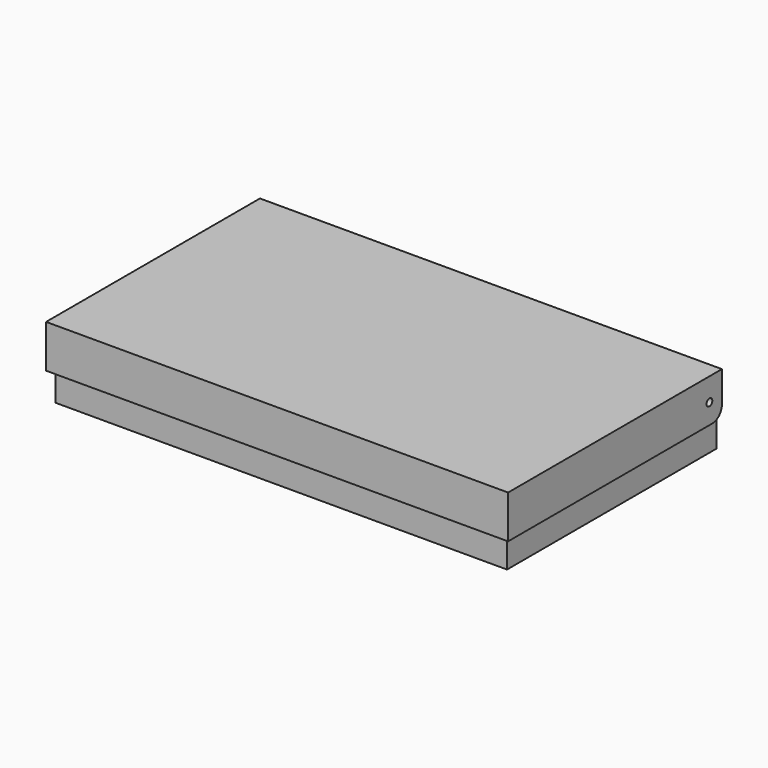
from build123d import *

# Parameters (mm, degrees)
F0_W          = 189.0018912738
F0_H          = 109.5
F0_W_2        = 25
F0_H_2        = 25
F1_DEPTH      = 25
F2_W          = 189.0018912738
F2_H          = 109.5
F3_DEPTH      = 2
F4_R          = 15
F6_DEPTH      = 3
F6_DEPTH_BACK = 15
F7_W          = 193.4018912738
F7_H          = 111.8995610192
F8_DEPTH      = 2
F9_T1_DEPTH   = 204.0018912738
F10_R         = 1.5
F11_DEPTH     = 200
F12_R         = 5


# Not quite as in the source:
# - a fillet or chamfer that OpenCascade refuses, or shapes differently, is made with other operations: its cross-section is extruded or revolved along the edge and cut away or added


with BuildPart() as f1:
    # F0 (on Top) → F1 (new body)
    with BuildSketch(Plane.XY):
        with Locations((79.4990543631, -39.75)):
            Rectangle(F0_W, F0_H)
        with Locations((0.0173321555, -79.5)):
            Rectangle(F0_W_2, F0_H_2, mode=Mode.SUBTRACT)
        with Locations((26.5173321555, -79.5)):
            Rectangle(F0_W_2, F0_H_2, mode=Mode.SUBTRACT)
        with Locations((53.0173321555, -79.5)):
            Rectangle(F0_W_2, F0_H_2, mode=Mode.SUBTRACT)
        with Locations((-0.0018912738, -53)):
            Rectangle(F0_W_2, F0_H_2, mode=Mode.SUBTRACT)
        with Locations((26.4981087262, -53)):
            Rectangle(F0_W_2, F0_H_2, mode=Mode.SUBTRACT)
        with Locations((52.9981087262, -53)):
            Rectangle(F0_W_2, F0_H_2, mode=Mode.SUBTRACT)
        with Locations((79.4981087262, -53)):
            Rectangle(F0_W_2, F0_H_2, mode=Mode.SUBTRACT)
        with Locations((79.5173321555, -79.5)):
            Rectangle(F0_W_2, F0_H_2, mode=Mode.SUBTRACT)
        with Locations((106.0173321555, -79.5)):
            Rectangle(F0_W_2, F0_H_2, mode=Mode.SUBTRACT)
        with Locations((132.5173321555, -79.5)):
            Rectangle(F0_W_2, F0_H_2, mode=Mode.SUBTRACT)
        with Locations((159.0173321555, -79.5)):
            Rectangle(F0_W_2, F0_H_2, mode=Mode.SUBTRACT)
        with Locations((105.9981087262, -53)):
            Rectangle(F0_W_2, F0_H_2, mode=Mode.SUBTRACT)
        with Locations((132.4981087262, -53)):
            Rectangle(F0_W_2, F0_H_2, mode=Mode.SUBTRACT)
        with Locations((158.9981087262, -53)):
            Rectangle(F0_W_2, F0_H_2, mode=Mode.SUBTRACT)
        with Locations((-0.0081907397, -26.5)):
            Rectangle(F0_W_2, F0_H_2, mode=Mode.SUBTRACT)
        with Locations((26.4918092603, -26.5)):
            Rectangle(F0_W_2, F0_H_2, mode=Mode.SUBTRACT)
        with Locations((52.9918092603, -26.5)):
            Rectangle(F0_W_2, F0_H_2, mode=Mode.SUBTRACT)
        with Locations((79.4918092603, -26.5)):
            Rectangle(F0_W_2, F0_H_2, mode=Mode.SUBTRACT)
        Rectangle(F0_W_2, F0_H_2, mode=Mode.SUBTRACT)
        with Locations((26.5, 0)):
            Rectangle(F0_W_2, F0_H_2, mode=Mode.SUBTRACT)
        with Locations((53, 0)):
            Rectangle(F0_W_2, F0_H_2, mode=Mode.SUBTRACT)
        with Locations((105.9918092603, -26.5)):
            Rectangle(F0_W_2, F0_H_2, mode=Mode.SUBTRACT)
        with Locations((132.4918092603, -26.5)):
            Rectangle(F0_W_2, F0_H_2, mode=Mode.SUBTRACT)
        with Locations((158.9918092603, -26.5)):
            Rectangle(F0_W_2, F0_H_2, mode=Mode.SUBTRACT)
        with Locations((79.5, 0)):
            Rectangle(F0_W_2, F0_H_2, mode=Mode.SUBTRACT)
        with Locations((106, 0)):
            Rectangle(F0_W_2, F0_H_2, mode=Mode.SUBTRACT)
        with Locations((132.5, 0)):
            Rectangle(F0_W_2, F0_H_2, mode=Mode.SUBTRACT)
        with Locations((159, 0)):
            Rectangle(F0_W_2, F0_H_2, mode=Mode.SUBTRACT)
    extrude(amount=F1_DEPTH)

    # F2 (on Top) → F3 (join)
    with BuildSketch(Plane.XY):
        with Locations((79.4990543631, -39.75)):
            Rectangle(F2_W, F2_H)
    extrude(amount=-F3_DEPTH)

    # F4
    f4_edges = [f1.edges().sort_by_distance(p)[0] for p in [
        (0, -12.5, 0),
        (26.5, -12.5, 0),
        (53, -12.5, 0),
        (79.5, -12.5, 0),
        (106, -12.5, 0),
        (132.5, -12.5, 0),
        (159, -12.5, 0),
        (-0.008191, -39, 0),
        (26.491809, -39, 0),
        (52.991809, -39, 0),
        (79.491809, -39, 0),
        (105.991809, -39, 0),
        (132.491809, -39, 0),
        (158.991809, -39, 0),
        (158.998109, -65.5, 0),
        (132.498109, -65.5, 0),
        (105.998109, -65.5, 0),
        (79.498109, -65.5, 0),
        (52.998109, -65.5, 0),
        (26.498109, -65.5, 0),
        (-0.001891, -65.5, 0),
        (0.017332, -92, 0),
        (26.517332, -92, 0),
        (53.017332, -92, 0),
        (79.517332, -92, 0),
        (106.017332, -92, 0),
        (132.517332, -92, 0),
        (159.017332, -92, 0),
    ]]
    fillet(f4_edges, radius=F4_R)

    # F9: fillet of radius 3 on 1 edges, made by hand

    # F9_s2 → F9_t1 (cut)
    with BuildSketch(Plane.YZ.offset(-22.5018912738)):
        with BuildLine():
            ThreePointArc((12, 25), (14.1213203436, 24.1213203436), (15, 22))
            Line((15, 22), (15, 25))
            Line((15, 25), (12, 25))
        make_face()
    extrude(amount=F9_T1_DEPTH, mode=Mode.SUBTRACT)


with BuildPart() as f6:
    # F5 (on face) → F6 (new body, two sides)
    with BuildSketch(Plane.XY.offset(25)) as f6_sk:
        Polygon((-15.2018912738, -94.7), (-15.2018912738, 15.1995610192), (-17.2018912738, 15.1995610192), (-17.2018912738, -96.7), (176.2, -96.7), (176.2, 15.1995610192), (174.2, 15.1995610192), (174.2, -94.7), align=None)
    extrude(amount=F6_DEPTH)
    extrude(f6_sk.sketch, amount=-F6_DEPTH_BACK)

    # F7 (on face) → F8 (join)
    with BuildSketch(Plane.XY.offset(28)):
        with Locations((79.4990543631, -40.7502194904)):
            Rectangle(F7_W, F7_H)
    extrude(amount=-F8_DEPTH)


with BuildPart() as f11_tool:
    # F10 (on face) → F11 (new body)
    with BuildSketch(Plane.YZ.offset(176.2)):
        with Locations((8.6607150733, 18.4004213661)):
            Circle(F10_R)
    extrude(amount=-F11_DEPTH)


with BuildPart() as f1_1:
    add(f1.part)

    # F11: cut by f11_tool
    add(f11_tool.part, mode=Mode.SUBTRACT)


with BuildPart() as f6_1:
    add(f6.part)

    # F11: cut by f11_tool
    add(f11_tool.part, mode=Mode.SUBTRACT)

    # F12
    f12_edges = [f6_1.edges().sort_by_distance(p)[0] for p in [
        (175.2, 15.199561, 10),
        (-16.201891, 15.199561, 10),
    ]]
    fillet(f12_edges, radius=F12_R)


solid = Compound([f1_1.part, f6_1.part])
